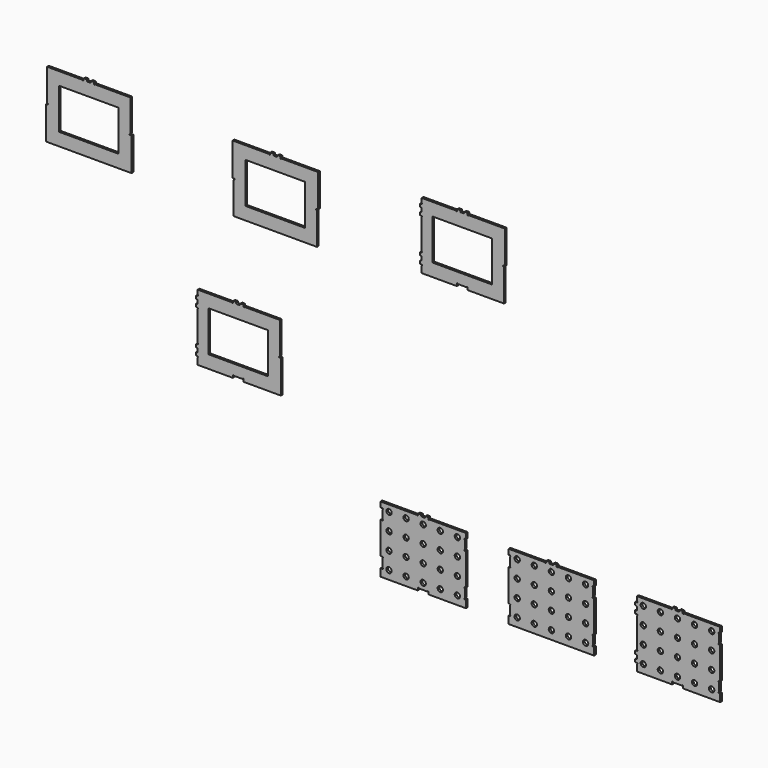
from build123d import *

# Parameters (mm, degrees)
F2_R     = 7.9375
F3_DEPTH = 6.35
F4_DEPTH = 6.35


# Not quite as in the source:
# - a variable given as a bare number and used for a length is read in inches; the dataset says mm whatever the document's units were


with BuildPart() as f3:
    # F2 (on Front) → F3 (new body)
    with BuildSketch(Plane.XZ):
        with BuildLine():
            Line((-869.4107007942, 91.9598769903), (-977.6147007942, 91.9598769903))
            Line((-977.6147007942, 91.9598769903), (-977.6147007942, 76.2118769903))
            Line((-977.6147007942, 76.2118769903), (-971.1377007942, 76.2118769903))
            ThreePointArc((-971.1377007942, 76.2118769903), (-969.604293545, 75.0352522244), (-970.3439507942, 73.2495616618))
            ThreePointArc((-970.3439507942, 73.2495616618), (-970.9250161227, 72.6684963333), (-971.1377007942, 71.8747463333))
            Line((-971.1377007942, 71.8747463333), (-971.1377007942, 48.5450076473))
            ThreePointArc((-971.1377007942, 48.5450076473), (-970.9250161227, 47.7512576473), (-970.3439507942, 47.1701923188))
            ThreePointArc((-970.3439507942, 47.1701923188), (-969.604293545, 45.3845017562), (-971.1377007942, 44.2078769903))
            Line((-971.1377007942, 44.2078769903), (-977.6147007942, 44.2078769903))
            Line((-977.6147007942, 44.2078769903), (-977.6147007942, -50.7881230097))
            Line((-977.6147007942, -50.7881230097), (-971.1377007942, -50.7881230097))
            ThreePointArc((-971.1377007942, -50.7881230097), (-969.604293545, -51.9647477756), (-970.3439507942, -53.7504383382))
            ThreePointArc((-970.3439507942, -53.7504383382), (-970.9250161227, -54.3315036667), (-971.1377007942, -55.1252536667))
            Line((-971.1377007942, -55.1252536667), (-971.1377007942, -78.4549923527))
            ThreePointArc((-971.1377007942, -78.4549923527), (-970.9250161227, -79.2487423527), (-970.3439507942, -79.8298076812))
            ThreePointArc((-970.3439507942, -79.8298076812), (-969.604293545, -81.6154982438), (-971.1377007942, -82.7921230097))
            Line((-971.1377007942, -82.7921230097), (-977.6147007942, -82.7921230097))
            Line((-977.6147007942, -82.7921230097), (-977.6147007942, -104.8901230097))
            Line((-977.6147007942, -104.8901230097), (-866.6167007942, -104.8901230097))
            Line((-866.6167007942, -104.8901230097), (-866.6167007942, -98.4131230097))
            ThreePointArc((-866.6167007942, -98.4131230097), (-865.4400760283, -96.8797157604), (-863.6543854657, -97.6193730097))
            ThreePointArc((-863.6543854657, -97.6193730097), (-863.0733201372, -98.2004383382), (-862.2795701372, -98.4131230097))
            Line((-862.2795701372, -98.4131230097), (-838.9498314512, -98.4131230097))
            ThreePointArc((-838.9498314512, -98.4131230097), (-838.1560814512, -98.2004383382), (-837.5750161227, -97.6193730097))
            ThreePointArc((-837.5750161227, -97.6193730097), (-835.7893255601, -96.8797157604), (-834.6127007942, -98.4131230097))
            Line((-834.6127007942, -98.4131230097), (-834.6127007942, -104.8901230097))
            Line((-834.6127007942, -104.8901230097), (-723.6147007942, -104.8901230097))
            Line((-723.6147007942, -104.8901230097), (-723.6147007942, -82.7921230097))
            Line((-723.6147007942, -82.7921230097), (-726.8532007942, -82.7921230097))
            ThreePointArc((-726.8532007942, -82.7921230097), (-728.3866080435, -81.6154982438), (-727.6469507942, -79.8298076812))
            ThreePointArc((-727.6469507942, -79.8298076812), (-727.0658854657, -79.2487423527), (-726.8532007942, -78.4549923527))
            Line((-726.8532007942, -78.4549923527), (-726.8532007942, -55.1252536667))
            ThreePointArc((-726.8532007942, -55.1252536667), (-727.0658854657, -54.3315036667), (-727.6469507942, -53.7504383382))
            ThreePointArc((-727.6469507942, -53.7504383382), (-728.3866080435, -51.9647477756), (-726.8532007942, -50.7881230097))
            Line((-726.8532007942, -50.7881230097), (-723.6147007942, -50.7881230097))
            Line((-723.6147007942, -50.7881230097), (-723.6147007942, 44.2078769903))
            Line((-723.6147007942, 44.2078769903), (-726.8532007942, 44.2078769903))
            ThreePointArc((-726.8532007942, 44.2078769903), (-728.3866080435, 45.3845017562), (-727.6469507942, 47.1701923188))
            ThreePointArc((-727.6469507942, 47.1701923188), (-727.0658854657, 47.7512576473), (-726.8532007942, 48.5450076473))
            Line((-726.8532007942, 48.5450076473), (-726.8532007942, 71.8747463333))
            ThreePointArc((-726.8532007942, 71.8747463333), (-727.0658854657, 72.6684963333), (-727.6469507942, 73.2495616618))
            ThreePointArc((-727.6469507942, 73.2495616618), (-728.3866080435, 75.0352522244), (-726.8532007942, 76.2118769903))
            Line((-726.8532007942, 76.2118769903), (-723.6147007942, 76.2118769903))
            Line((-723.6147007942, 76.2118769903), (-723.6147007942, 91.9598769903))
            Line((-723.6147007942, 91.9598769903), (-831.8187007942, 91.9598769903))
            ThreePointArc((-831.8187007942, 91.9598769903), (-833.4062007942, 90.3723769903), (-834.9937007942, 91.9598769903))
            Line((-834.9937007942, 91.9598769903), (-834.9937007942, 95.4523769903))
            ThreePointArc((-834.9937007942, 95.4523769903), (-835.4586687791, 96.5749090054), (-836.5812007942, 97.0398769903))
            Line((-836.5812007942, 97.0398769903), (-843.1852007942, 97.0398769903))
            ThreePointArc((-843.1852007942, 97.0398769903), (-844.3077328094, 96.5749090054), (-844.7727007942, 95.4523769903))
            Line((-844.7727007942, 95.4523769903), (-844.7727007942, 93.5473769903))
            ThreePointArc((-844.7727007942, 93.5473769903), (-845.2376687791, 92.4248449752), (-846.3602007942, 91.9598769903))
            Line((-846.3602007942, 91.9598769903), (-850.6147007942, 91.9598769903))
            Line((-850.6147007942, 91.9598769903), (-854.8692007942, 91.9598769903))
            ThreePointArc((-854.8692007942, 91.9598769903), (-855.9917328094, 92.4248449752), (-856.4567007942, 93.5473769903))
            Line((-856.4567007942, 93.5473769903), (-856.4567007942, 95.4523769903))
            ThreePointArc((-856.4567007942, 95.4523769903), (-856.9216687791, 96.5749090054), (-858.0442007942, 97.0398769903))
            Line((-858.0442007942, 97.0398769903), (-864.6482007942, 97.0398769903))
            ThreePointArc((-864.6482007942, 97.0398769903), (-865.7707328094, 96.5749090054), (-866.2357007942, 95.4523769903))
            Line((-866.2357007942, 95.4523769903), (-866.2357007942, 91.9598769903))
            ThreePointArc((-866.2357007942, 91.9598769903), (-867.8232007942, 90.3723769903), (-869.4107007942, 91.9598769903))
        make_face()
        with Locations((-952.2147007942, -79.4901230097)):
            Circle(F2_R, mode=Mode.SUBTRACT)
        with Locations((-901.4147007942, -79.4901230097)):
            Circle(F2_R, mode=Mode.SUBTRACT)
        with Locations((-850.6147007942, -79.4901230097)):
            Circle(F2_R, mode=Mode.SUBTRACT)
        with Locations((-799.8147007942, -79.4901230097)):
            Circle(F2_R, mode=Mode.SUBTRACT)
        with Locations((-749.0147007942, -79.4901230097)):
            Circle(F2_R, mode=Mode.SUBTRACT)
        with Locations((-952.2147007942, -28.6901230097)):
            Circle(F2_R, mode=Mode.SUBTRACT)
        with Locations((-901.4147007942, -28.6901230097)):
            Circle(F2_R, mode=Mode.SUBTRACT)
        with Locations((-850.6147007942, -28.6901230097)):
            Circle(F2_R, mode=Mode.SUBTRACT)
        with Locations((-952.2147007942, 22.1098769903)):
            Circle(F2_R, mode=Mode.SUBTRACT)
        with Locations((-901.4147007942, 22.1098769903)):
            Circle(F2_R, mode=Mode.SUBTRACT)
        with Locations((-850.6147007942, 22.1098769903)):
            Circle(F2_R, mode=Mode.SUBTRACT)
        with Locations((-799.8147007942, -28.6901230097)):
            Circle(F2_R, mode=Mode.SUBTRACT)
        with Locations((-749.0147007942, -28.6901230097)):
            Circle(F2_R, mode=Mode.SUBTRACT)
        with Locations((-799.8147007942, 22.1098769903)):
            Circle(F2_R, mode=Mode.SUBTRACT)
        with Locations((-749.0147007942, 22.1098769903)):
            Circle(F2_R, mode=Mode.SUBTRACT)
        with Locations((-952.2147007942, 72.9098769903)):
            Circle(F2_R, mode=Mode.SUBTRACT)
        with Locations((-901.4147007942, 72.9098769903)):
            Circle(F2_R, mode=Mode.SUBTRACT)
        with Locations((-850.6147007942, 72.9098769903)):
            Circle(F2_R, mode=Mode.SUBTRACT)
        with Locations((-799.8147007942, 72.9098769903)):
            Circle(F2_R, mode=Mode.SUBTRACT)
        with Locations((-749.0147007942, 72.9098769903)):
            Circle(F2_R, mode=Mode.SUBTRACT)
    extrude(amount=F3_DEPTH)


with BuildPart() as f3b:
    # F2 (on Front) → F3, piece 2 (new body)
    with BuildSketch(Plane.XZ):
        with BuildLine():
            Line((-488.4107007942, 91.9598769903), (-596.6147007942, 91.9598769903))
            Line((-596.6147007942, 91.9598769903), (-596.6147007942, 76.2118769903))
            Line((-596.6147007942, 76.2118769903), (-593.3762007942, 76.2118769903))
            ThreePointArc((-593.3762007942, 76.2118769903), (-591.842793545, 75.0352522244), (-592.5824507942, 73.2495616618))
            ThreePointArc((-592.5824507942, 73.2495616618), (-593.1635161227, 72.6684963333), (-593.3762007942, 71.8747463333))
            Line((-593.3762007942, 71.8747463333), (-593.3762007942, 48.5450076473))
            ThreePointArc((-593.3762007942, 48.5450076473), (-593.1635161227, 47.7512576473), (-592.5824507942, 47.1701923188))
            ThreePointArc((-592.5824507942, 47.1701923188), (-591.842793545, 45.3845017562), (-593.3762007942, 44.2078769903))
            Line((-593.3762007942, 44.2078769903), (-596.6147007942, 44.2078769903))
            Line((-596.6147007942, 44.2078769903), (-596.6147007942, -50.7881230097))
            Line((-596.6147007942, -50.7881230097), (-593.3762007942, -50.7881230097))
            ThreePointArc((-593.3762007942, -50.7881230097), (-591.842793545, -51.9647477756), (-592.5824507942, -53.7504383382))
            ThreePointArc((-592.5824507942, -53.7504383382), (-593.1635161227, -54.3315036667), (-593.3762007942, -55.1252536667))
            Line((-593.3762007942, -55.1252536667), (-593.3762007942, -78.4549923527))
            ThreePointArc((-593.3762007942, -78.4549923527), (-593.1635161227, -79.2487423527), (-592.5824507942, -79.8298076812))
            ThreePointArc((-592.5824507942, -79.8298076812), (-591.842793545, -81.6154982438), (-593.3762007942, -82.7921230097))
            Line((-593.3762007942, -82.7921230097), (-596.6147007942, -82.7921230097))
            Line((-596.6147007942, -82.7921230097), (-596.6147007942, -104.8901230097))
            Line((-596.6147007942, -104.8901230097), (-342.6147007942, -104.8901230097))
            Line((-342.6147007942, -104.8901230097), (-342.6147007942, -82.7921230097))
            Line((-342.6147007942, -82.7921230097), (-345.8532007942, -82.7921230097))
            ThreePointArc((-345.8532007942, -82.7921230097), (-347.3866080435, -81.6154982438), (-346.6469507942, -79.8298076812))
            ThreePointArc((-346.6469507942, -79.8298076812), (-346.0658854657, -79.2487423527), (-345.8532007942, -78.4549923527))
            Line((-345.8532007942, -78.4549923527), (-345.8532007942, -55.1252536667))
            ThreePointArc((-345.8532007942, -55.1252536667), (-346.0658854657, -54.3315036667), (-346.6469507942, -53.7504383382))
            ThreePointArc((-346.6469507942, -53.7504383382), (-347.3866080435, -51.9647477756), (-345.8532007942, -50.7881230097))
            Line((-345.8532007942, -50.7881230097), (-342.6147007942, -50.7881230097))
            Line((-342.6147007942, -50.7881230097), (-342.6147007942, 44.2078769903))
            Line((-342.6147007942, 44.2078769903), (-345.8532007942, 44.2078769903))
            ThreePointArc((-345.8532007942, 44.2078769903), (-347.3866080435, 45.3845017562), (-346.6469507942, 47.1701923188))
            ThreePointArc((-346.6469507942, 47.1701923188), (-346.0658854657, 47.7512576473), (-345.8532007942, 48.5450076473))
            Line((-345.8532007942, 48.5450076473), (-345.8532007942, 71.8747463333))
            ThreePointArc((-345.8532007942, 71.8747463333), (-346.0658854657, 72.6684963333), (-346.6469507942, 73.2495616618))
            ThreePointArc((-346.6469507942, 73.2495616618), (-347.3866080435, 75.0352522244), (-345.8532007942, 76.2118769903))
            Line((-345.8532007942, 76.2118769903), (-342.6147007942, 76.2118769903))
            Line((-342.6147007942, 76.2118769903), (-342.6147007942, 91.9598769903))
            Line((-342.6147007942, 91.9598769903), (-450.8187007942, 91.9598769903))
            ThreePointArc((-450.8187007942, 91.9598769903), (-452.4062007942, 90.3723769903), (-453.9937007942, 91.9598769903))
            Line((-453.9937007942, 91.9598769903), (-453.9937007942, 95.4523769903))
            ThreePointArc((-453.9937007942, 95.4523769903), (-454.4586687791, 96.5749090055), (-455.5812007942, 97.0398769903))
            Line((-455.5812007942, 97.0398769903), (-462.1852007942, 97.0398769903))
            ThreePointArc((-462.1852007942, 97.0398769903), (-463.3077328094, 96.5749090055), (-463.7727007942, 95.4523769903))
            Line((-463.7727007942, 95.4523769903), (-463.7727007942, 93.5473769903))
            ThreePointArc((-463.7727007942, 93.5473769903), (-464.2376687791, 92.4248449752), (-465.3602007942, 91.9598769903))
            Line((-465.3602007942, 91.9598769903), (-469.6147007942, 91.9598769903))
            Line((-469.6147007942, 91.9598769903), (-473.8692007942, 91.9598769903))
            ThreePointArc((-473.8692007942, 91.9598769903), (-474.9917328094, 92.4248449752), (-475.4567007942, 93.5473769903))
            Line((-475.4567007942, 93.5473769903), (-475.4567007942, 95.4523769903))
            ThreePointArc((-475.4567007942, 95.4523769903), (-475.9216687791, 96.5749090055), (-477.0442007942, 97.0398769903))
            Line((-477.0442007942, 97.0398769903), (-483.6482007942, 97.0398769903))
            ThreePointArc((-483.6482007942, 97.0398769903), (-484.7707328094, 96.5749090055), (-485.2357007942, 95.4523769903))
            Line((-485.2357007942, 95.4523769903), (-485.2357007942, 91.9598769903))
            ThreePointArc((-485.2357007942, 91.9598769903), (-486.8232007942, 90.3723769903), (-488.4107007942, 91.9598769903))
        make_face()
        with Locations((-571.2147007942, -79.4901230097)):
            Circle(F2_R, mode=Mode.SUBTRACT)
        with Locations((-520.4147007942, -79.4901230097)):
            Circle(F2_R, mode=Mode.SUBTRACT)
        with Locations((-469.6147007942, -79.4901230097)):
            Circle(F2_R, mode=Mode.SUBTRACT)
        with Locations((-571.2147007942, -28.6901230097)):
            Circle(F2_R, mode=Mode.SUBTRACT)
        with Locations((-520.4147007942, -28.6901230097)):
            Circle(F2_R, mode=Mode.SUBTRACT)
        with Locations((-469.6147007942, -28.6901230097)):
            Circle(F2_R, mode=Mode.SUBTRACT)
        with Locations((-571.2147007942, 22.1098769903)):
            Circle(F2_R, mode=Mode.SUBTRACT)
        with Locations((-520.4147007942, 22.1098769903)):
            Circle(F2_R, mode=Mode.SUBTRACT)
        with Locations((-469.6147007942, 22.1098769903)):
            Circle(F2_R, mode=Mode.SUBTRACT)
        with Locations((-571.2147007942, 72.9098769903)):
            Circle(F2_R, mode=Mode.SUBTRACT)
        with Locations((-520.4147007942, 72.9098769903)):
            Circle(F2_R, mode=Mode.SUBTRACT)
        with Locations((-469.6147007942, 72.9098769903)):
            Circle(F2_R, mode=Mode.SUBTRACT)
        with Locations((-418.8147007942, -79.4901230097)):
            Circle(F2_R, mode=Mode.SUBTRACT)
        with Locations((-368.0147007942, -79.4901230097)):
            Circle(F2_R, mode=Mode.SUBTRACT)
        with Locations((-418.8147007942, -28.6901230097)):
            Circle(F2_R, mode=Mode.SUBTRACT)
        with Locations((-368.0147007942, -28.6901230097)):
            Circle(F2_R, mode=Mode.SUBTRACT)
        with Locations((-418.8147007942, 22.1098769903)):
            Circle(F2_R, mode=Mode.SUBTRACT)
        with Locations((-368.0147007942, 22.1098769903)):
            Circle(F2_R, mode=Mode.SUBTRACT)
        with Locations((-418.8147007942, 72.9098769903)):
            Circle(F2_R, mode=Mode.SUBTRACT)
        with Locations((-368.0147007942, 72.9098769903)):
            Circle(F2_R, mode=Mode.SUBTRACT)
    extrude(amount=F3_DEPTH)


with BuildPart() as f3c:
    # F2 (on Front) → F3, piece 3 (new body)
    with BuildSketch(Plane.XZ):
        with BuildLine():
            Line((-113.7607007942, 91.9598769903), (-215.6147007942, 91.9598769903))
            Line((-215.6147007942, 91.9598769903), (-215.6147007942, 79.0058769836))
            ThreePointArc((-215.6147007942, 79.0058769836), (-214.0272007942, 77.4183769836), (-215.6147007942, 75.8308769836))
            Line((-215.6147007942, 75.8308769836), (-219.1072007942, 75.8308769836))
            ThreePointArc((-219.1072007942, 75.8308769836), (-220.2297328094, 75.3659089987), (-220.6947007942, 74.2433769836))
            Line((-220.6947007942, 74.2433769836), (-220.6947007942, 67.6393769836))
            ThreePointArc((-220.6947007942, 67.6393769836), (-220.2297328094, 66.5168449685), (-219.1072007942, 66.0518769836))
            Line((-219.1072007942, 66.0518769836), (-217.2022008332, 66.0518769836))
            ThreePointArc((-217.2022008332, 66.0518769836), (-216.0796688232, 65.5869090039), (-215.6147008332, 64.4643769982))
            Line((-215.6147008332, 64.4643769982), (-215.6147007942, 60.2098769903))
            Line((-215.6147007942, 60.2098769903), (-215.6147007972, 55.9553769825))
            ThreePointArc((-215.6147007972, 55.9553769825), (-216.0796687825, 54.8328449681), (-217.2022007972, 54.3678769836))
            Line((-217.2022007972, 54.3678769836), (-219.1072007942, 54.3678769836))
            ThreePointArc((-219.1072007942, 54.3678769836), (-220.2297328094, 53.9029089987), (-220.6947007942, 52.7803769836))
            Line((-220.6947007942, 52.7803769836), (-220.6947007942, 46.1763769836))
            ThreePointArc((-220.6947007942, 46.1763769836), (-220.2297328094, 45.0538449685), (-219.1072007942, 44.5888769836))
            Line((-219.1072007942, 44.5888769836), (-215.6147007942, 44.5888769836))
            ThreePointArc((-215.6147007942, 44.5888769836), (-214.0272007942, 43.0013769836), (-215.6147007942, 41.4138769836))
            Line((-215.6147007942, 41.4138769836), (-215.6147007942, -47.9941230099))
            ThreePointArc((-215.6147007942, -47.9941230099), (-214.0272007942, -49.5816230099), (-215.6147007942, -51.1691230099))
            Line((-215.6147007942, -51.1691230099), (-219.1072007942, -51.1691230099))
            ThreePointArc((-219.1072007942, -51.1691230099), (-220.2297328093, -51.6340909948), (-220.6947007942, -52.7566230099))
            Line((-220.6947007942, -52.7566230099), (-220.6947007942, -59.3606230099))
            ThreePointArc((-220.6947007942, -59.3606230099), (-220.2297328093, -60.483155025), (-219.1072007942, -60.9481230099))
            Line((-219.1072007942, -60.9481230099), (-217.2022007954, -60.9481230099))
            ThreePointArc((-217.2022007954, -60.9481230099), (-216.0796687804, -61.4130909946), (-215.6147007954, -62.5356230095))
            Line((-215.6147007954, -62.5356230095), (-215.6147007942, -66.7901230097))
            Line((-215.6147007942, -66.7901230097), (-215.6147007942, -71.0446230099))
            ThreePointArc((-215.6147007942, -71.0446230099), (-216.0796687791, -72.167155025), (-217.2022007942, -72.6321230099))
            Line((-217.2022007942, -72.6321230099), (-219.1072007942, -72.6321230099))
            ThreePointArc((-219.1072007942, -72.6321230099), (-220.2297328093, -73.0970909948), (-220.6947007942, -74.2196230099))
            Line((-220.6947007942, -74.2196230099), (-220.6947007942, -80.8236230099))
            ThreePointArc((-220.6947007942, -80.8236230099), (-220.2297328094, -81.946155025), (-219.1072007942, -82.4111230099))
            Line((-219.1072007942, -82.4111230099), (-215.6147007942, -82.4111230099))
            ThreePointArc((-215.6147007942, -82.4111230099), (-214.0272007942, -83.9986230099), (-215.6147007942, -85.5861230099))
            Line((-215.6147007942, -85.5861230099), (-215.6147007942, -104.8901230097))
            Line((-215.6147007942, -104.8901230097), (-110.9667007942, -104.8901230097))
            Line((-110.9667007942, -104.8901230097), (-110.9667007942, -98.4131230097))
            ThreePointArc((-110.9667007942, -98.4131230097), (-109.7900760283, -96.8797157604), (-108.0043854657, -97.6193730097))
            ThreePointArc((-108.0043854657, -97.6193730097), (-107.4233201372, -98.2004383382), (-106.6295701372, -98.4131230097))
            Line((-106.6295701372, -98.4131230097), (-83.2998314512, -98.4131230097))
            ThreePointArc((-83.2998314512, -98.4131230097), (-82.5060814512, -98.2004383382), (-81.9250161227, -97.6193730097))
            ThreePointArc((-81.9250161227, -97.6193730097), (-80.1393255601, -96.8797157604), (-78.9627007942, -98.4131230097))
            Line((-78.9627007942, -98.4131230097), (-78.9627007942, -104.8901230097))
            Line((-78.9627007942, -104.8901230097), (32.0352992058, -104.8901230097))
            Line((32.0352992058, -104.8901230097), (32.0352992058, -82.7921230097))
            Line((32.0352992058, -82.7921230097), (28.7967992058, -82.7921230097))
            ThreePointArc((28.7967992058, -82.7921230097), (27.2633919565, -81.6154982438), (28.0030492058, -79.8298076812))
            ThreePointArc((28.0030492058, -79.8298076812), (28.5841145343, -79.2487423527), (28.7967992058, -78.4549923527))
            Line((28.7967992058, -78.4549923527), (28.7967992058, -55.1252536667))
            ThreePointArc((28.7967992058, -55.1252536667), (28.5841145343, -54.3315036667), (28.0030492058, -53.7504383382))
            ThreePointArc((28.0030492058, -53.7504383382), (27.2633919565, -51.9647477756), (28.7967992058, -50.7881230097))
            Line((28.7967992058, -50.7881230097), (32.0352992058, -50.7881230097))
            Line((32.0352992058, -50.7881230097), (32.0352992058, 44.2078769903))
            Line((32.0352992058, 44.2078769903), (28.7967992058, 44.2078769903))
            ThreePointArc((28.7967992058, 44.2078769903), (27.2633919565, 45.3845017562), (28.0030492058, 47.1701923188))
            ThreePointArc((28.0030492058, 47.1701923188), (28.5841145343, 47.7512576473), (28.7967992058, 48.5450076473))
            Line((28.7967992058, 48.5450076473), (28.7967992058, 71.8747463333))
            ThreePointArc((28.7967992058, 71.8747463333), (28.5841145343, 72.6684963333), (28.0030492058, 73.2495616618))
            ThreePointArc((28.0030492058, 73.2495616618), (27.2633919565, 75.0352522244), (28.7967992058, 76.2118769903))
            Line((28.7967992058, 76.2118769903), (32.0352992058, 76.2118769903))
            Line((32.0352992058, 76.2118769903), (32.0352992058, 91.9598769903))
            Line((32.0352992058, 91.9598769903), (-76.1687007942, 91.9598769903))
            ThreePointArc((-76.1687007942, 91.9598769903), (-77.7562007942, 90.3723769903), (-79.3437007942, 91.9598769903))
            Line((-79.3437007942, 91.9598769903), (-79.3437007942, 95.4523769903))
            ThreePointArc((-79.3437007942, 95.4523769903), (-79.8086687791, 96.5749090055), (-80.9312007942, 97.0398769903))
            Line((-80.9312007942, 97.0398769903), (-87.5352007942, 97.0398769903))
            ThreePointArc((-87.5352007942, 97.0398769903), (-88.6577328094, 96.5749090055), (-89.1227007942, 95.4523769903))
            Line((-89.1227007942, 95.4523769903), (-89.1227007942, 93.5473769903))
            ThreePointArc((-89.1227007942, 93.5473769903), (-89.5876687791, 92.4248449752), (-90.7102007942, 91.9598769903))
            Line((-90.7102007942, 91.9598769903), (-94.9647007942, 91.9598769903))
            Line((-94.9647007942, 91.9598769903), (-99.2192007942, 91.9598769903))
            ThreePointArc((-99.2192007942, 91.9598769903), (-100.3417328094, 92.4248449752), (-100.8067007942, 93.5473769903))
            Line((-100.8067007942, 93.5473769903), (-100.8067007942, 95.4523769903))
            ThreePointArc((-100.8067007942, 95.4523769903), (-101.2716687791, 96.5749090055), (-102.3942007942, 97.0398769903))
            Line((-102.3942007942, 97.0398769903), (-108.9982007942, 97.0398769903))
            ThreePointArc((-108.9982007942, 97.0398769903), (-110.1207328094, 96.5749090055), (-110.5857007942, 95.4523769903))
            Line((-110.5857007942, 95.4523769903), (-110.5857007942, 91.9598769903))
            ThreePointArc((-110.5857007942, 91.9598769903), (-112.1732007942, 90.3723769903), (-113.7607007942, 91.9598769903))
        make_face()
        with Locations((-196.5647007942, -79.4901230097)):
            Circle(F2_R, mode=Mode.SUBTRACT)
        with Locations((-145.7647007942, -79.4901230097)):
            Circle(F2_R, mode=Mode.SUBTRACT)
        with Locations((-94.9647007942, -79.4901230097)):
            Circle(F2_R, mode=Mode.SUBTRACT)
        with Locations((-44.1647007942, -79.4901230097)):
            Circle(F2_R, mode=Mode.SUBTRACT)
        with Locations((6.6352992058, -79.4901230097)):
            Circle(F2_R, mode=Mode.SUBTRACT)
        with Locations((-196.5647007942, -28.6901230097)):
            Circle(F2_R, mode=Mode.SUBTRACT)
        with Locations((-145.7647007942, -28.6901230097)):
            Circle(F2_R, mode=Mode.SUBTRACT)
        with Locations((-94.9647007942, -28.6901230097)):
            Circle(F2_R, mode=Mode.SUBTRACT)
        with Locations((-196.5647007942, 22.1098769903)):
            Circle(F2_R, mode=Mode.SUBTRACT)
        with Locations((-145.7647007942, 22.1098769903)):
            Circle(F2_R, mode=Mode.SUBTRACT)
        with Locations((-94.9647007942, 22.1098769903)):
            Circle(F2_R, mode=Mode.SUBTRACT)
        with Locations((-44.1647007942, -28.6901230097)):
            Circle(F2_R, mode=Mode.SUBTRACT)
        with Locations((6.6352992058, -28.6901230097)):
            Circle(F2_R, mode=Mode.SUBTRACT)
        with Locations((-44.1647007942, 22.1098769903)):
            Circle(F2_R, mode=Mode.SUBTRACT)
        with Locations((6.6352992058, 22.1098769903)):
            Circle(F2_R, mode=Mode.SUBTRACT)
        with Locations((-196.5647007942, 72.9098769903)):
            Circle(F2_R, mode=Mode.SUBTRACT)
        with Locations((-145.7647007942, 72.9098769903)):
            Circle(F2_R, mode=Mode.SUBTRACT)
        with Locations((-94.9647007942, 72.9098769903)):
            Circle(F2_R, mode=Mode.SUBTRACT)
        with Locations((-44.1647007942, 72.9098769903)):
            Circle(F2_R, mode=Mode.SUBTRACT)
        with Locations((6.6352992058, 72.9098769903)):
            Circle(F2_R, mode=Mode.SUBTRACT)
    extrude(amount=F3_DEPTH)


with BuildPart() as f4:
    # F2 (on Front) → F4 (new body)
    with BuildSketch(Plane.XZ):
        with BuildLine():
            Line((-1863.0483950106, 907.0695124176), (-1968.0138950106, 907.0695124176))
            Line((-1968.0138950106, 907.0695124176), (-1968.0138950106, 813.1530124175))
            ThreePointArc((-1968.0138950106, 813.1530124175), (-1967.5489270258, 812.0304804024), (-1966.4263950106, 811.5655124175))
            ThreePointArc((-1966.4263950106, 811.5655124175), (-1964.8388950106, 809.9780124175), (-1966.4263950106, 808.3905124175))
            Line((-1966.4263950106, 808.3905124175), (-1971.2523950106, 808.3905124175))
            Line((-1971.2523950106, 808.3905124175), (-1971.2523950106, 710.2195124176))
            Line((-1971.2523950106, 710.2195124176), (-1717.2523950106, 710.2195124176))
            Line((-1717.2523950106, 710.2195124176), (-1717.2523950106, 808.3905124176))
            Line((-1717.2523950106, 808.3905124176), (-1722.0783950106, 808.3905124176))
            ThreePointArc((-1722.0783950106, 808.3905124176), (-1723.6658950106, 809.9780124176), (-1722.0783950106, 811.5655124176))
            ThreePointArc((-1722.0783950106, 811.5655124176), (-1720.9558629955, 812.0304804024), (-1720.4908950106, 813.1530124176))
            Line((-1720.4908950106, 813.1530124176), (-1720.4908950106, 907.0695124176))
            Line((-1720.4908950106, 907.0695124176), (-1825.4563950106, 907.0695124176))
            ThreePointArc((-1825.4563950106, 907.0695124176), (-1827.0438950106, 905.4820124176), (-1828.6313950106, 907.0695124176))
            Line((-1828.6313950106, 907.0695124176), (-1828.6313950106, 910.5620124176))
            ThreePointArc((-1828.6313950106, 910.5620124176), (-1829.0963629955, 911.6845444327), (-1830.2188950106, 912.1495124176))
            Line((-1830.2188950106, 912.1495124176), (-1836.8228950106, 912.1495124176))
            ThreePointArc((-1836.8228950106, 912.1495124176), (-1837.9454270258, 911.6845444327), (-1838.4103950106, 910.5620124176))
            Line((-1838.4103950106, 910.5620124176), (-1838.4103950106, 908.6570124176))
            ThreePointArc((-1838.4103950106, 908.6570124176), (-1838.8753629955, 907.5344804024), (-1839.9978950106, 907.0695124176))
            Line((-1839.9978950106, 907.0695124176), (-1844.2523950106, 907.0695124176))
            Line((-1844.2523950106, 907.0695124176), (-1848.5068950106, 907.0695124176))
            ThreePointArc((-1848.5068950106, 907.0695124176), (-1849.6294270258, 907.5344804024), (-1850.0943950106, 908.6570124176))
            Line((-1850.0943950106, 908.6570124176), (-1850.0943950106, 910.5620124176))
            ThreePointArc((-1850.0943950106, 910.5620124176), (-1850.5593629955, 911.6845444327), (-1851.6818950106, 912.1495124176))
            Line((-1851.6818950106, 912.1495124176), (-1858.2858950106, 912.1495124176))
            ThreePointArc((-1858.2858950106, 912.1495124176), (-1859.4084270258, 911.6845444327), (-1859.8733950106, 910.5620124176))
            Line((-1859.8733950106, 910.5620124176), (-1859.8733950106, 907.0695124176))
            ThreePointArc((-1859.8733950106, 907.0695124176), (-1861.4608950106, 905.4820124176), (-1863.0483950106, 907.0695124176))
        make_face()
        with BuildLine():
            ThreePointArc((-1933.1523950106, 867.3820124176), (-1932.6874270258, 868.5045444327), (-1931.5648950106, 868.9695124176))
            Line((-1931.5648950106, 868.9695124176), (-1756.9398950106, 868.9695124176))
            ThreePointArc((-1756.9398950106, 868.9695124176), (-1755.8173629955, 868.5045444327), (-1755.3523950106, 867.3820124176))
            Line((-1755.3523950106, 867.3820124176), (-1755.3523950106, 749.9070124176))
            ThreePointArc((-1755.3523950106, 749.9070124176), (-1755.8173629955, 748.7844804024), (-1756.9398950106, 748.3195124176))
            Line((-1756.9398950106, 748.3195124176), (-1931.5648950106, 748.3195124176))
            ThreePointArc((-1931.5648950106, 748.3195124176), (-1932.6874270258, 748.7844804024), (-1933.1523950106, 749.9070124176))
            Line((-1933.1523950106, 749.9070124176), (-1933.1523950106, 867.3820124176))
        make_face(mode=Mode.SUBTRACT)
    extrude(amount=F4_DEPTH)


with BuildPart() as f4b:
    # F2 (on Front) → F4, piece 2 (new body)
    with BuildSketch(Plane.XZ):
        with BuildLine():
            Line((-1419.112892319, 469.4469458482), (-1520.966892319, 469.4469458482))
            Line((-1520.966892319, 469.4469458482), (-1520.966892319, 456.4928377227))
            ThreePointArc((-1520.966892319, 456.4928377227), (-1519.379392319, 454.9053377227), (-1520.966892319, 453.3178377227))
            Line((-1520.966892319, 453.3178377227), (-1524.4592926576, 453.3178377227))
            ThreePointArc((-1524.4592926576, 453.3178377227), (-1525.5818226798, 452.8528717308), (-1526.0467926576, 451.7303433596))
            Line((-1526.0467926576, 451.7303433596), (-1526.0468161074, 445.1263433597))
            ThreePointArc((-1526.0468161074, 445.1263433597), (-1525.5818501155, 444.0038077005), (-1524.4593161074, 443.5388377227))
            Line((-1524.4593161074, 443.5388377227), (-1522.5546431972, 443.5388377227))
            ThreePointArc((-1522.5546431972, 443.5388377227), (-1521.4321442796, 443.0739028344), (-1520.9671432, 441.9514313353))
            Line((-1520.9671432, 441.9514313353), (-1520.966892319, 437.6969458482))
            Line((-1520.966892319, 437.6969458482), (-1520.9665636351, 433.4424603663))
            ThreePointArc((-1520.9665636351, 433.4424603663), (-1521.431488255, 432.3198490694), (-1522.5540636304, 431.8548377226))
            Line((-1522.5540636304, 431.8548377226), (-1524.4593688693, 431.8548377226))
            ThreePointArc((-1524.4593688693, 431.8548377226), (-1525.5818988914, 431.3898717307), (-1526.0468688693, 430.2673433596))
            Line((-1526.0468688693, 430.2673433596), (-1526.046892319, 423.6633433596))
            ThreePointArc((-1526.046892319, 423.6633433596), (-1525.5819263271, 422.5408077005), (-1524.459392319, 422.0758377227))
            Line((-1524.459392319, 422.0758377227), (-1520.966892319, 422.0758377227))
            ThreePointArc((-1520.966892319, 422.0758377227), (-1519.379392319, 420.4883377227), (-1520.966892319, 418.9008377227))
            Line((-1520.966892319, 418.9008377227), (-1520.966892319, 329.4929711906))
            ThreePointArc((-1520.966892319, 329.4929711906), (-1519.379392319, 327.9054711906), (-1520.966892319, 326.3179711906))
            Line((-1520.966892319, 326.3179711906), (-1524.4578037095, 326.3179711906))
            ThreePointArc((-1524.4578037095, 326.3179711906), (-1525.5803277462, 325.8530111842), (-1526.0453037094, 324.7304937571))
            Line((-1526.0453037094, 324.7304937571), (-1526.0453975859, 318.1264937578))
            ThreePointArc((-1526.0453975859, 318.1264937578), (-1525.5804375797, 317.0039471546), (-1524.4578975861, 316.5389711913))
            Line((-1524.4578975861, 316.5389711913), (-1522.5543149909, 316.5389711913))
            ThreePointArc((-1522.5543149909, 316.5389711913), (-1521.4317727745, 316.073993005), (-1520.9668149912, 314.9514423376))
            Line((-1520.9668149912, 314.9514423376), (-1520.966892319, 310.6969458482))
            Line((-1520.966892319, 310.6969458482), (-1520.9669508274, 306.4424493584))
            ThreePointArc((-1520.9669508274, 306.4424493584), (-1521.4319265308, 305.3199314562), (-1522.5544508273, 304.8549711899))
            Line((-1522.5544508273, 304.8549711899), (-1524.4581088084, 304.8549711899))
            ThreePointArc((-1524.4581088084, 304.8549711899), (-1525.580632845, 304.3900111835), (-1526.0456088082, 303.2674937564))
            Line((-1526.0456088082, 303.2674937564), (-1526.0457026848, 296.6634937571))
            ThreePointArc((-1526.0457026848, 296.6634937571), (-1525.5807426785, 295.540947154), (-1524.458202685, 295.0759711906))
            Line((-1524.458202685, 295.0759711906), (-1520.966892319, 295.0759711906))
            ThreePointArc((-1520.966892319, 295.0759711906), (-1519.379392319, 293.4884711906), (-1520.966892319, 291.9009711906))
            Line((-1520.966892319, 291.9009711906), (-1520.966892319, 272.5969458482))
            Line((-1520.966892319, 272.5969458482), (-1416.318892319, 272.5969458482))
            Line((-1416.318892319, 272.5969458482), (-1416.318892319, 279.0739458481))
            ThreePointArc((-1416.318892319, 279.0739458481), (-1415.1422675531, 280.6073530974), (-1413.3565769905, 279.8676958481))
            ThreePointArc((-1413.3565769905, 279.8676958481), (-1412.775511662, 279.2866305196), (-1411.981761662, 279.0739458481))
            Line((-1411.981761662, 279.0739458481), (-1388.652022976, 279.0739458481))
            ThreePointArc((-1388.652022976, 279.0739458481), (-1387.858272976, 279.2866305196), (-1387.2772076475, 279.8676958481))
            ThreePointArc((-1387.2772076475, 279.8676958482), (-1385.4915170849, 280.6073530974), (-1384.314892319, 279.0739458481))
            Line((-1384.314892319, 279.0739458481), (-1384.314892319, 272.5969458482))
            Line((-1384.314892319, 272.5969458482), (-1273.316892319, 272.5969458482))
            Line((-1273.316892319, 272.5969458482), (-1273.316892319, 370.7679458482))
            Line((-1273.316892319, 370.7679458482), (-1278.142892319, 370.7679458482))
            ThreePointArc((-1278.142892319, 370.7679458482), (-1279.730392319, 372.3554458482), (-1278.142892319, 373.9429458482))
            ThreePointArc((-1278.142892319, 373.9429458482), (-1277.0203603039, 374.407913833), (-1276.555392319, 375.5304458482))
            Line((-1276.555392319, 375.5304458482), (-1276.555392319, 469.4469458482))
            Line((-1276.555392319, 469.4469458482), (-1381.520892319, 469.4469458482))
            ThreePointArc((-1381.520892319, 469.4469458482), (-1383.108392319, 467.8594458482), (-1384.695892319, 469.4469458482))
            Line((-1384.695892319, 469.4469458482), (-1384.695892319, 472.9394458481))
            ThreePointArc((-1384.695892319, 472.9394458481), (-1385.1608603039, 474.0619778633), (-1386.283392319, 474.5269458481))
            Line((-1386.283392319, 474.5269458481), (-1392.887392319, 474.5269458481))
            ThreePointArc((-1392.887392319, 474.5269458481), (-1394.0099243341, 474.0619778633), (-1394.474892319, 472.9394458481))
            Line((-1394.474892319, 472.9394458481), (-1394.474892319, 471.0344458482))
            ThreePointArc((-1394.474892319, 471.0344458482), (-1394.9398603039, 469.911913833), (-1396.062392319, 469.4469458482))
            Line((-1396.062392319, 469.4469458482), (-1400.316892319, 469.4469458482))
            Line((-1400.316892319, 469.4469458482), (-1404.571392319, 469.4469458482))
            ThreePointArc((-1404.571392319, 469.4469458482), (-1405.6939243341, 469.911913833), (-1406.158892319, 471.0344458482))
            Line((-1406.158892319, 471.0344458482), (-1406.158892319, 472.9394458481))
            ThreePointArc((-1406.158892319, 472.9394458481), (-1406.6238603039, 474.0619778633), (-1407.746392319, 474.5269458481))
            Line((-1407.746392319, 474.5269458481), (-1414.350392319, 474.5269458481))
            ThreePointArc((-1414.350392319, 474.5269458481), (-1415.4729243341, 474.0619778633), (-1415.937892319, 472.9394458481))
            Line((-1415.937892319, 472.9394458481), (-1415.937892319, 469.4469458482))
            ThreePointArc((-1415.937892319, 469.4469458482), (-1417.525392319, 467.8594458482), (-1419.112892319, 469.4469458482))
        make_face()
        with BuildLine():
            ThreePointArc((-1489.216892319, 429.7594458482), (-1488.7519243341, 430.8819778633), (-1487.629392319, 431.3469458482))
            Line((-1487.629392319, 431.3469458482), (-1313.004392319, 431.3469458482))
            ThreePointArc((-1313.004392319, 431.3469458482), (-1311.8818603039, 430.8819778633), (-1311.416892319, 429.7594458482))
            Line((-1311.416892319, 429.7594458482), (-1311.416892319, 312.2844458482))
            ThreePointArc((-1311.416892319, 312.2844458482), (-1311.8818603039, 311.161913833), (-1313.004392319, 310.6969458482))
            Line((-1313.004392319, 310.6969458482), (-1487.629392319, 310.6969458482))
            ThreePointArc((-1487.629392319, 310.6969458482), (-1488.7519243341, 311.161913833), (-1489.216892319, 312.2844458482))
            Line((-1489.216892319, 312.2844458482), (-1489.216892319, 429.7594458482))
        make_face(mode=Mode.SUBTRACT)
    extrude(amount=F4_DEPTH)


with BuildPart() as f4c:
    # F2 (on Front) → F4, piece 3 (new body)
    with BuildSketch(Plane.XZ):
        with BuildLine():
            Line((-1308.866048867, 893.3399084899), (-1417.070048867, 893.3399084899))
            Line((-1417.070048867, 893.3399084899), (-1417.070048867, 795.1689084899))
            Line((-1417.070048867, 795.1689084899), (-1412.244048867, 795.1689084899))
            ThreePointArc((-1412.244048867, 795.1689084899), (-1410.656548867, 793.5814084899), (-1412.244048867, 791.9939084899))
            ThreePointArc((-1412.244048867, 791.9939084899), (-1413.3665808821, 791.528940505), (-1413.831548867, 790.4064084899))
            Line((-1413.831548867, 790.4064084899), (-1413.831548867, 696.4899084899))
            Line((-1413.831548867, 696.4899084899), (-1166.308548867, 696.4899084899))
            Line((-1166.308548867, 696.4899084899), (-1166.308548867, 790.4064084899))
            ThreePointArc((-1166.308548867, 790.4064084899), (-1166.7735168519, 791.528940505), (-1167.896048867, 791.9939084899))
            ThreePointArc((-1167.896048867, 791.9939084899), (-1169.483548867, 793.5814084899), (-1167.896048867, 795.1689084899))
            Line((-1167.896048867, 795.1689084899), (-1163.070048867, 795.1689084899))
            Line((-1163.070048867, 795.1689084899), (-1163.070048867, 893.3399084899))
            Line((-1163.070048867, 893.3399084899), (-1271.274048867, 893.3399084899))
            ThreePointArc((-1271.274048867, 893.3399084899), (-1272.861548867, 891.7524084899), (-1274.449048867, 893.3399084899))
            Line((-1274.449048867, 893.3399084899), (-1274.449048867, 896.8324084899))
            ThreePointArc((-1274.449048867, 896.8324084899), (-1274.9140168519, 897.954940505), (-1276.036548867, 898.4199084899))
            Line((-1276.036548867, 898.4199084899), (-1282.640548867, 898.4199084899))
            ThreePointArc((-1282.640548867, 898.4199084899), (-1283.7630808822, 897.954940505), (-1284.228048867, 896.8324084899))
            Line((-1284.228048867, 896.8324084899), (-1284.228048867, 894.9274084899))
            ThreePointArc((-1284.228048867, 894.9274084899), (-1284.6930168519, 893.8048764747), (-1285.815548867, 893.3399084899))
            Line((-1285.815548867, 893.3399084899), (-1290.070048867, 893.3399084899))
            Line((-1290.070048867, 893.3399084899), (-1294.324548867, 893.3399084899))
            ThreePointArc((-1294.324548867, 893.3399084899), (-1295.4470808821, 893.8048764747), (-1295.912048867, 894.9274084899))
            Line((-1295.912048867, 894.9274084899), (-1295.912048867, 896.8324084899))
            ThreePointArc((-1295.912048867, 896.8324084899), (-1296.3770168519, 897.954940505), (-1297.499548867, 898.4199084899))
            Line((-1297.499548867, 898.4199084899), (-1304.103548867, 898.4199084899))
            ThreePointArc((-1304.103548867, 898.4199084899), (-1305.2260808821, 897.954940505), (-1305.691048867, 896.8324084899))
            Line((-1305.691048867, 896.8324084899), (-1305.691048867, 893.3399084899))
            ThreePointArc((-1305.691048867, 893.3399084899), (-1307.278548867, 891.7524084899), (-1308.866048867, 893.3399084899))
        make_face()
        with BuildLine():
            ThreePointArc((-1378.970048867, 853.6524084899), (-1378.5050808821, 854.774940505), (-1377.382548867, 855.2399084899))
            Line((-1377.382548867, 855.2399084899), (-1202.757548867, 855.2399084899))
            ThreePointArc((-1202.757548867, 855.2399084899), (-1201.6350168519, 854.774940505), (-1201.170048867, 853.6524084899))
            Line((-1201.170048867, 853.6524084899), (-1201.170048867, 736.1774084899))
            ThreePointArc((-1201.170048867, 736.1774084899), (-1201.6350168519, 735.0548764747), (-1202.757548867, 734.5899084899))
            Line((-1202.757548867, 734.5899084899), (-1377.382548867, 734.5899084899))
            ThreePointArc((-1377.382548867, 734.5899084899), (-1378.5050808821, 735.0548764747), (-1378.970048867, 736.1774084899))
            Line((-1378.970048867, 736.1774084899), (-1378.970048867, 853.6524084899))
        make_face(mode=Mode.SUBTRACT)
    extrude(amount=F4_DEPTH)


with BuildPart() as f4d:
    # F2 (on Front) → F4, piece 4 (new body)
    with BuildSketch(Plane.XZ):
        with BuildLine():
            Line((-753.1852057565, 925.9708392645), (-855.0392057565, 925.9708392645))
            Line((-855.0392057565, 925.9708392645), (-855.0392057565, 913.016731139))
            ThreePointArc((-855.0392057565, 913.016731139), (-853.4517057565, 911.429231139), (-855.0392057565, 909.841731139))
            Line((-855.0392057565, 909.841731139), (-858.531606095, 909.841731139))
            ThreePointArc((-858.531606095, 909.841731139), (-859.6541361172, 909.3767651471), (-860.119106095, 908.2542367759))
            Line((-860.119106095, 908.2542367759), (-860.1191295448, 901.650236776))
            ThreePointArc((-860.1191295448, 901.650236776), (-859.6541635529, 900.5277011169), (-858.5316295448, 900.062731139))
            Line((-858.5316295448, 900.062731139), (-856.6269566418, 900.062731139))
            ThreePointArc((-856.6269566418, 900.062731139), (-855.5044577251, 899.5977962517), (-855.0394566445, 898.4753247543))
            Line((-855.0394566445, 898.4753247543), (-855.0392057565, 894.2208392657))
            Line((-855.0392057565, 894.2208392657), (-855.0388770728, 889.9663537825))
            ThreePointArc((-855.0388770728, 889.9663537825), (-855.5038016928, 888.8437424857), (-856.6263770681, 888.3787311389))
            Line((-856.6263770681, 888.3787311389), (-858.5316823067, 888.3787311389))
            ThreePointArc((-858.5316823067, 888.3787311389), (-859.6542123289, 887.913765147), (-860.1191823067, 886.7912367759))
            Line((-860.1191823067, 886.7912367759), (-860.1192057565, 880.1872367759))
            ThreePointArc((-860.1192057565, 880.1872367759), (-859.6542397646, 879.0647011168), (-858.5317057565, 878.599731139))
            Line((-858.5317057565, 878.599731139), (-855.0392057565, 878.599731139))
            ThreePointArc((-855.0392057565, 878.599731139), (-853.4517057565, 877.012231139), (-855.0392057565, 875.424731139))
            Line((-855.0392057565, 875.424731139), (-855.0392057565, 786.0168646069))
            ThreePointArc((-855.0392057565, 786.0168646069), (-853.4517057565, 784.4293646069), (-855.0392057565, 782.8418646069))
            Line((-855.0392057565, 782.8418646069), (-858.530117147, 782.8418646069))
            ThreePointArc((-858.530117147, 782.8418646069), (-859.6526411836, 782.3769046005), (-860.1176171468, 781.2543871734))
            Line((-860.1176171468, 781.2543871734), (-860.1177110234, 774.650387174))
            ThreePointArc((-860.1177110234, 774.6503871741), (-859.6527510171, 773.5278405709), (-858.5302110236, 773.0628646076))
            Line((-858.5302110236, 773.0628646076), (-856.6266284285, 773.0628646076))
            ThreePointArc((-856.6266284285, 773.0628646076), (-855.5040862121, 772.5978864213), (-855.0391284288, 771.4753357539))
            Line((-855.0391284288, 771.4753357539), (-855.0392057565, 767.2208392645))
            Line((-855.0392057565, 767.2208392645), (-855.0392642647, 762.9663427748))
            ThreePointArc((-855.0392642647, 762.9663427748), (-855.5042399681, 761.8438248725), (-856.6267642646, 761.3788646062))
            Line((-856.6267642646, 761.3788646062), (-858.5304222459, 761.3788646062))
            ThreePointArc((-858.5304222459, 761.3788646062), (-859.6529462825, 760.9139045998), (-860.1179222457, 759.7913871727))
            Line((-860.1179222457, 759.7913871727), (-860.1180161223, 753.1873871734))
            ThreePointArc((-860.1180161223, 753.1873871734), (-859.653056116, 752.0648405703), (-858.5305161225, 751.5998646069))
            Line((-858.5305161225, 751.5998646069), (-855.0392057565, 751.5998646069))
            ThreePointArc((-855.0392057565, 751.5998646069), (-853.4517057565, 750.0123646069), (-855.0392057565, 748.4248646069))
            Line((-855.0392057565, 748.4248646069), (-855.0392057565, 729.1208392645))
            Line((-855.0392057565, 729.1208392645), (-750.3912057565, 729.1208392645))
            Line((-750.3912057565, 729.1208392645), (-750.3912057565, 735.5978392645))
            ThreePointArc((-750.3912057565, 735.5978392645), (-749.2145809906, 737.1312465137), (-747.428890428, 736.3915892645))
            ThreePointArc((-747.428890428, 736.3915892645), (-746.8478250995, 735.810523936), (-746.0540750995, 735.5978392645))
            Line((-746.0540750995, 735.5978392645), (-722.7243364135, 735.5978392645))
            ThreePointArc((-722.7243364135, 735.5978392645), (-721.9305864135, 735.810523936), (-721.349521085, 736.3915892645))
            ThreePointArc((-721.349521085, 736.3915892645), (-719.5638305224, 737.1312465137), (-718.3872057565, 735.5978392645))
            Line((-718.3872057565, 735.5978392645), (-718.3872057565, 729.1208392645))
            Line((-718.3872057565, 729.1208392645), (-610.6277057565, 729.1208392645))
            Line((-610.6277057565, 729.1208392645), (-610.6277057565, 823.0373392645))
            ThreePointArc((-610.6277057565, 823.0373392645), (-611.0926737414, 824.1598712796), (-612.2152057565, 824.6248392645))
            ThreePointArc((-612.2152057565, 824.6248392645), (-613.8027057565, 826.2123392645), (-612.2152057565, 827.7998392645))
            Line((-612.2152057565, 827.7998392645), (-607.3892057565, 827.7998392645))
            Line((-607.3892057565, 827.7998392645), (-607.3892057565, 925.9708392645))
            Line((-607.3892057565, 925.9708392645), (-715.5932057565, 925.9708392645))
            ThreePointArc((-715.5932057565, 925.9708392645), (-717.1807057565, 924.3833392645), (-718.7682057565, 925.9708392645))
            Line((-718.7682057565, 925.9708392645), (-718.7682057565, 929.4633392645))
            ThreePointArc((-718.7682057565, 929.4633392645), (-719.2331737414, 930.5858712796), (-720.3557057565, 931.0508392645))
            Line((-720.3557057565, 931.0508392645), (-726.9597057565, 931.0508392645))
            ThreePointArc((-726.9597057565, 931.0508392645), (-728.0822377717, 930.5858712796), (-728.5472057565, 929.4633392645))
            Line((-728.5472057565, 929.4633392645), (-728.5472057565, 927.5583392645))
            ThreePointArc((-728.5472057565, 927.5583392645), (-729.0121737414, 926.4358072494), (-730.1347057565, 925.9708392645))
            Line((-730.1347057565, 925.9708392645), (-734.3892057565, 925.9708392645))
            Line((-734.3892057565, 925.9708392645), (-738.6437057565, 925.9708392645))
            ThreePointArc((-738.6437057565, 925.9708392645), (-739.7662377716, 926.4358072494), (-740.2312057565, 927.5583392645))
            Line((-740.2312057565, 927.5583392645), (-740.2312057565, 929.4633392645))
            ThreePointArc((-740.2312057565, 929.4633392645), (-740.6961737414, 930.5858712796), (-741.8187057565, 931.0508392645))
            Line((-741.8187057565, 931.0508392645), (-748.4227057565, 931.0508392645))
            ThreePointArc((-748.4227057565, 931.0508392645), (-749.5452377716, 930.5858712796), (-750.0102057565, 929.4633392645))
            Line((-750.0102057565, 929.4633392645), (-750.0102057565, 925.9708392645))
            ThreePointArc((-750.0102057565, 925.9708392645), (-751.5977057565, 924.3833392645), (-753.1852057565, 925.9708392645))
        make_face()
        with BuildLine():
            ThreePointArc((-823.2892057565, 886.2833392645), (-822.8242377716, 887.4058712796), (-821.7017057565, 887.8708392645))
            Line((-821.7017057565, 887.8708392645), (-647.0767057565, 887.8708392645))
            ThreePointArc((-647.0767057565, 887.8708392645), (-645.9541737414, 887.4058712796), (-645.4892057565, 886.2833392645))
            Line((-645.4892057565, 886.2833392645), (-645.4892057565, 768.8083392645))
            ThreePointArc((-645.4892057565, 768.8083392645), (-645.9541737414, 767.6858072494), (-647.0767057565, 767.2208392645))
            Line((-647.0767057565, 767.2208392645), (-821.7017057565, 767.2208392645))
            ThreePointArc((-821.7017057565, 767.2208392645), (-822.8242377716, 767.6858072494), (-823.2892057565, 768.8083392645))
            Line((-823.2892057565, 768.8083392645), (-823.2892057565, 886.2833392645))
        make_face(mode=Mode.SUBTRACT)
    extrude(amount=F4_DEPTH)


solid = Compound([f3.part, f3b.part, f3c.part, f4.part, f4b.part, f4c.part, f4d.part])
